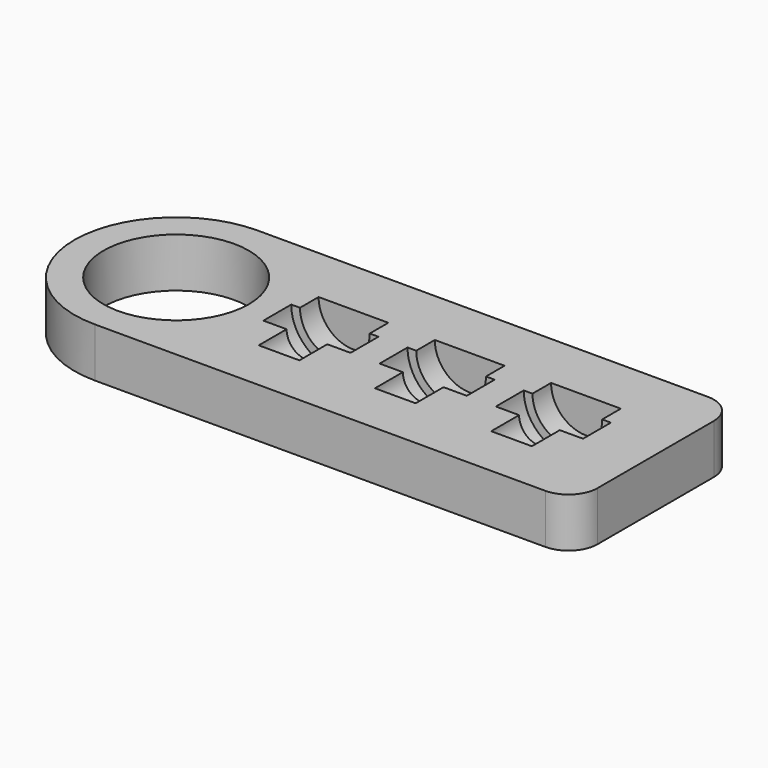
from build123d import *

# Parameters (mm, degrees)
F0_R         = 12.5
F1_DEPTH     = 8.5
F6_TEXT_SIZE = 5.5555555556
F7_DEPTH     = 1


# Not quite as in the source:
# - Text() gives the source's letters only with a copy of the font that has no kerning and outlines rounded to 1/6400 em; it was checked with that copy


with BuildPart() as f1:
    # F0 (on Top) → F1 (new body)
    with BuildSketch(Plane.XY):
        with BuildLine():
            ThreePointArc((0, 17.5), (5.1256313292, 5.1256313292), (17.5, 0))
            Line((17.5, 0), (95, 0))
            ThreePointArc((95, 0), (98.5355339059, 1.4644660941), (100, 5))
            Line((100, 5), (100, 30))
            ThreePointArc((100, 30), (98.5355339059, 33.5355339059), (95, 35))
            Line((95, 35), (17.5, 35))
            ThreePointArc((17.5, 35), (5.1256313292, 29.8743686708), (0, 17.5))
        make_face()
        with Locations((17.5, 17.5)):
            Circle(F0_R, mode=Mode.SUBTRACT)
    extrude(amount=F1_DEPTH)

    # F2 (on face) → F3 (revolve, cut)
    with BuildSketch(Plane.XY.offset(8.5)):
        Polygon((42, 15), (42, 9), (45.5, 9), (45.5, 15), (49.5, 15), (49.5, 21), (48, 21), (48, 25), (42, 25), (42, 21), align=None)
    revolve(axis=Axis((42, 18, 8.5), (0, 1, 0)), mode=Mode.SUBTRACT)

    # F2 (on face) → F4 (revolve, cut)
    with BuildSketch(Plane.XY.offset(8.5)):
        Polygon((62, 15), (62, 9), (65.5, 9), (65.5, 15), (69.5, 15), (69.5, 21), (68, 21), (68, 25), (62, 25), (62, 21), align=None)
    revolve(axis=Axis((62, 18, 8.5), (0, 1, 0)), mode=Mode.SUBTRACT)

    # F2 (on face) → F5 (revolve, cut)
    with BuildSketch(Plane.XY.offset(8.5)):
        Polygon((82, 15), (82, 9), (85.5, 9), (85.5, 15), (89.5, 15), (89.5, 21), (88, 21), (88, 25), (82, 25), (82, 21), align=None)
    revolve(axis=Axis((82, 18, 8.5), (0, 1, 0)), mode=Mode.SUBTRACT)

    # F6 (on face) → F7 (cut)
    with BuildSketch(Plane(origin=(0, 0, 0), x_dir=(1, 0, 0), z_dir=(0, 0, -1))):
        with Locations((30, -9)):
            Text('835', F6_TEXT_SIZE, font='Open Sans', text_align=(TextAlign.LEFT, TextAlign.BOTTOM))
    extrude(amount=-F7_DEPTH, mode=Mode.SUBTRACT)


solid = f1.part
